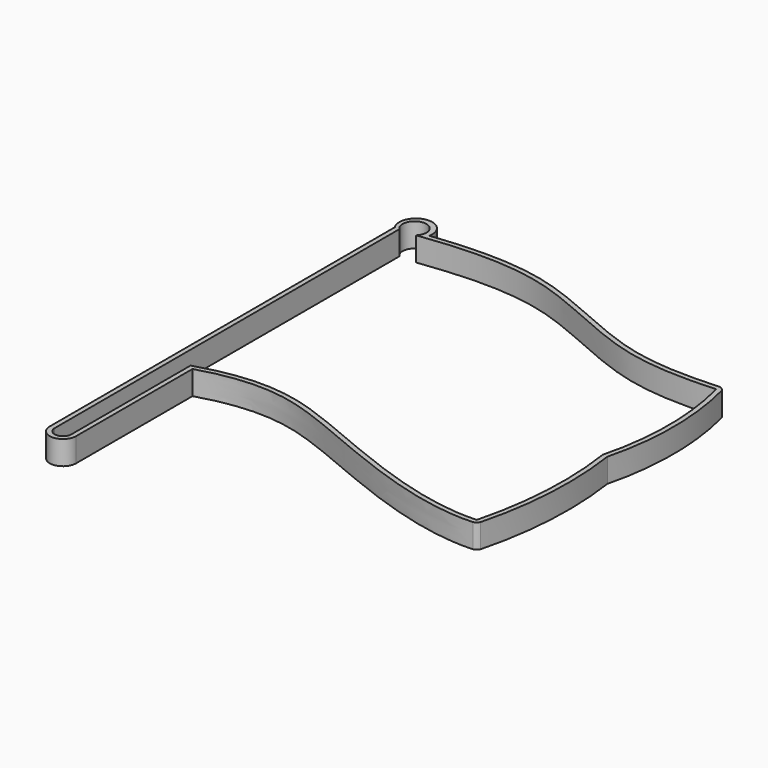
from build123d import *

# Parameters (mm, degrees)
F1_DEPTH = 10


# Not quite as in the source:
# - ends of sketch curves that miss each other by under 0.0002 mm in the source are joined
# - the dataset's text gives a spline's control points without its knots; the knots are read off the source's solid


with BuildPart() as f1:
    # F0 (on Top) → F1 (new body)
    with BuildSketch(Plane.XY):
        with BuildLine():
            add(Edge.make_bspline(
                [(-32.0717603685, 90.6650278101), (-22.6072106937, 91.7771953124), (-10.0475440841, 92.4848849696), (3.6956683451, 91.6771338871), (13.1587032628, 90.1554889027), (20.177912997, 88.2814250809), (25.4905952659, 86.5018265315), (29.3783079521, 85.048524055), (33.2317351771, 83.4964897914), (37.0847322841, 81.8683634163), (40.9309796698, 80.1950073854), (46.0522129373, 77.9423684419), (52.4380412295, 75.1597143213), (60.0687375349, 72.1067767095), (66.3886490848, 69.9915144149), (71.4168091625, 68.6710870322), (76.4711447666, 67.5865600883), (82.8830745584, 66.6447010226), (90.8928692935, 66.0944561137), (99.3734539828, 66.044221184), (105.4415076167, 66.2904204014), (108.6031889873, 66.4697045451)],
                knots=[0.0144163887, 0.0144163887, 0.0144163887, 0.0144163887, 0.125, 0.1875, 0.25, 0.3125, 0.34375, 0.375, 0.40625, 0.4375, 0.46875, 0.5, 0.5625, 0.625, 0.6875, 0.71875, 0.75, 0.8125, 0.875, 0.9375, 0.9999857998, 0.9999857998, 0.9999857998, 0.9999857998], degree=3))
            ThreePointArc((-32.0717603685, 90.6650278101), (-40.11542792, 98.8491939294), (-44.588655293, 88.2817103021))
            Line((-44.588655293, 88.2817103021), (-44.588655293, -91.751370728))
            ThreePointArc((-44.588655293, -91.751370728), (-39.1257780595, -97.3252437628), (-33.588655293, -91.825120151))
            Line((-33.588655293, -91.825120151), (-33.588655293, -31.0750725633))
            add(Edge.make_bspline(
                [(-33.588655293, -31.0750725633), (-29.7598616278, -29.8946681081), (-22.1331621407, -28.0403330655), (-11.9070299186, -26.9484905638), (-2.6613936601, -27.2941093305), (4.091968927, -28.4689975989), (9.029928343, -29.7426320734), (12.5267586359, -30.8158903572), (15.289178389, -31.7679005158), (17.4222340695, -32.5392521166), (19.500765876, -33.3086566138), (22.0175912224, -34.2733243973), (25.9571914454, -35.8423186295), (30.8792798676, -37.8892805467), (36.2209357083, -40.1473205581), (40.9916460511, -42.1341346297), (44.8854514537, -43.7309490338), (49.1332502268, -45.4350402842), (55.1917813533, -47.7841707939), (63.3954819264, -50.7595347383), (73.8797915494, -54.0433373779), (84.6442178433, -56.6923398623), (95.3365110676, -58.3540175883), (102.190233253, -58.5612355822), (105.4932190717, -58.3739154882)],
                knots=[0.0066837565, 0.0066837565, 0.0066837565, 0.0066837565, 0.0625, 0.125, 0.1875, 0.25, 0.28125, 0.3125, 0.34375, 0.359375, 0.375, 0.40625, 0.4375, 0.5, 0.5625, 0.59375, 0.625, 0.65625, 0.6875, 0.75, 0.8125, 0.875, 0.9375, 1, 1, 1, 1], degree=3))
            ThreePointArc((105.4932190717, -58.3739154882), (106.5097720026, -57.7560035228), (107.3155141735, -56.8808037672))
            ThreePointArc((107.3155141735, -56.8808037672), (112.1296667517, -26.0756479033), (110.7553929349, 5.0731091236))
            ThreePointArc((110.7553929349, 5.0731091236), (114.4672074111, 35.0459508708), (110.6468217034, 65.0051474915))
            ThreePointArc((110.6468217034, 65.0051474915), (109.7571071585, 65.9217599682), (108.6031889873, 66.4697045451))
        make_face()
        with BuildLine():
            ThreePointArc((-35.588655293, -91.7870268215), (-39.088655293, -95.2870268215), (-42.588655293, -91.7870268215))
            Line((-42.588655293, -91.7870268215), (-42.588655293, 88.2129731785))
            ThreePointArc((-42.588655293, 88.2129731785), (-40.9939696433, 96.3142265766), (-34.1257211905, 91.7315971859))
            ThreePointArc((-34.1257211905, 91.7315971859), (-34.5060259023, 89.8262828356), (-35.588655293, 88.2129731785))
            add(Edge.make_bspline(
                [(-35.588655293, 88.2129731785), (-1.1016856227, 92.7182770236), (26.7916774552, 85.7840012678), (67.9249790647, 64.5181886354), (93.1049781144, 63.5875508402), (108.7185872682, 64.4730353366)],
                knots=[0, 0, 0, 0, 0.3897948797, 0.6934169356, 1, 1, 1, 1], degree=3))
            ThreePointArc((108.7185872682, 64.4730353366), (112.4674061228, 34.8265703154), (108.7185872682, 5.1801052942))
            ThreePointArc((108.7185872682, 5.1801052942), (110.1436326512, -25.7663342367), (105.3799763325, -56.3771240414))
            add(Edge.make_bspline(
                [(-35.588655293, -29.6091232449), (-10.5246130655, -21.5155236612), (17.1593937874, -29.4044774674), (43.6188962482, -41.5787762466), (85.8071658515, -57.4871441567), (105.3799763325, -56.3771240414)],
                knots=[0, 0, 0, 0, 0.3537827801, 0.6156755201, 1, 1, 1, 1], degree=3))
            Line((-35.588655293, -29.6091232449), (-35.588655293, -91.7870268215))
        make_face(mode=Mode.SUBTRACT)
    extrude(amount=F1_DEPTH)


solid = f1.part
